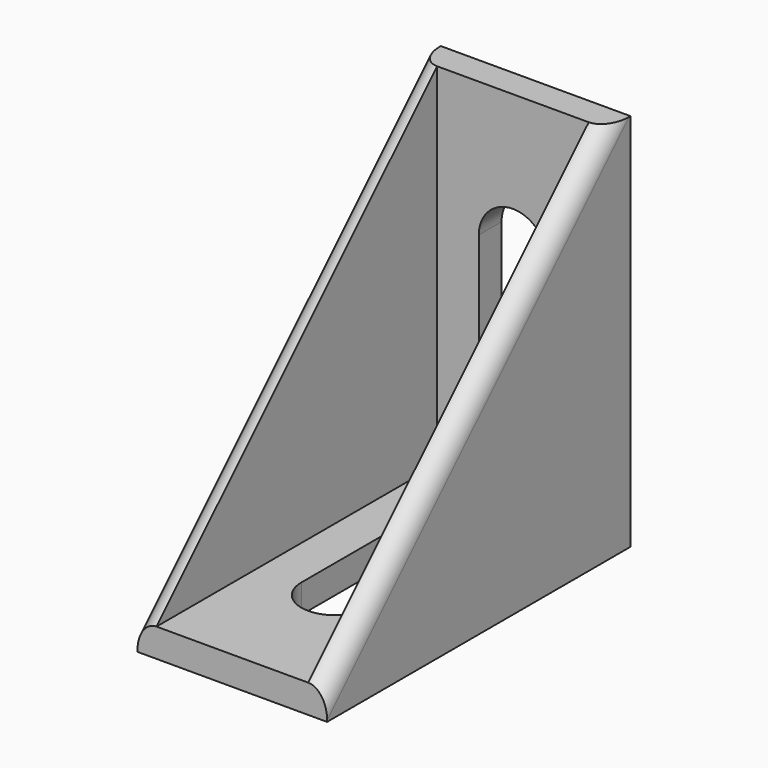
from build123d import *

# Parameters (mm, degrees)
F0_W     = 10
F0_H     = 20
F1_DEPTH = 1.5
F2_W     = 10
F2_H     = 1.5
F3_DEPTH = 18.5
F5_DEPTH = 1.501
F7_DEPTH = 1.501
F9_DEPTH = 1
F10_R    = 0.99999


# Not quite as in the source:
# - a fillet or chamfer is up to 0.001 mm smaller than in the source, because OpenCascade refuses the exact size
# - a pattern or mirror of a feature is missing from the dataset's text; its kind, count and spacing are read off the source's solid


with BuildPart() as f1:
    # F0 (on Top) → F1 (new body)
    with BuildSketch(Plane.XY):
        Rectangle(F0_W, F0_H)
    extrude(amount=F1_DEPTH)

    # F2 (on face) → F3 (join)
    with BuildSketch(Plane.XY.offset(1.5)):
        with Locations((0, 9.25)):
            Rectangle(F2_W, F2_H)
    extrude(amount=F3_DEPTH)

    # F4 (on face) → F5 (cut, through all)
    with BuildSketch(Plane.XY.offset(1.5)):
        with BuildLine():
            ThreePointArc((0, -5), (1.2727922061, -4.4727922061), (1.8, -3.2))
            Line((1.8, -3.2), (1.8, 3.2))
            ThreePointArc((1.8, 3.2), (1.2727922061, 4.4727922061), (0, 5))
            ThreePointArc((0, 5), (-1.2727922061, 4.4727922061), (-1.8, 3.2))
            Line((-1.8, 3.2), (-1.8, -3.2))
            ThreePointArc((-1.8, -3.2), (-1.2727922061, -4.4727922061), (0, -5))
        make_face()
    extrude(amount=-F5_DEPTH, mode=Mode.SUBTRACT)

    # F6 (on face) → F7 (cut, through all)
    with BuildSketch(Plane.XZ.offset(-8.5)):
        with BuildLine():
            ThreePointArc((0, 4.6788305809), (1.2727922061, 5.2060383747), (1.8, 6.4788305809))
            Line((1.8, 6.4788305809), (1.8, 12.8788305809))
            ThreePointArc((1.8, 12.8788305809), (1.2727922061, 14.151622787), (0, 14.6788305809))
            ThreePointArc((0, 14.6788305809), (-1.2727922061, 14.151622787), (-1.8, 12.8788305809))
            Line((-1.8, 12.8788305809), (-1.8, 6.4788305809))
            ThreePointArc((-1.8, 6.4788305809), (-1.2727922061, 5.2060383747), (0, 4.6788305809))
        make_face()
    extrude(amount=-F7_DEPTH, mode=Mode.SUBTRACT)

    # F8 (on face) → F9 (join)
    with BuildSketch(Plane(origin=(-5, 0, 0), x_dir=(0, -1, 0), z_dir=(-1, 0, 0))):
        Polygon((10, 1.5), (-8.5, 20), (-8.5, 1.5), align=None)
    f9 = extrude(amount=-F9_DEPTH)

    # F9_copies: F9 across plane
    add(f9.mirror(Plane(origin=(0, 0, 0), x_dir=(0, 0, 1), z_dir=(1, 0, 0))))

    # F10 (radius 1 in the source; OpenCascade refuses exactly that, so slightly less here)
    f10_edges = [f1.edges().sort_by_distance(p)[0] for p in [
        (-5, -0.75, 10.75),
        (5, -0.75, 10.75),
    ]]
    fillet(f10_edges, radius=F10_R)


solid = f1.part
